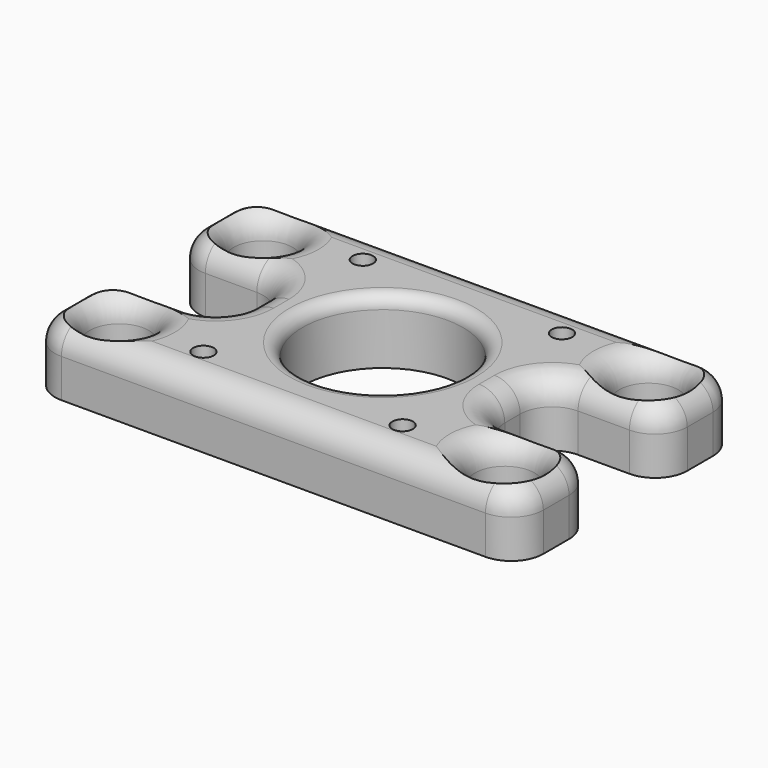
from build123d import *

# Parameters (mm, degrees)
F1_W          = 40
F1_H          = 43
F2_DEPTH      = 10
F3_R          = 12.5
F3_R_2        = 1.6
F4_DEPTH      = 10.001
F5_W          = 18
F5_H          = 15
F5_R          = 2.6
F6_DEPTH      = 10
F7_R          = 5
F8_R          = 4.6
F8_R_2        = 2.6
F9_DEPTH      = 7
F10_T1_DEPTH  = 66
F10_T3_DEPTH  = 3
F10_T5_DEPTH  = 8
F10_T7_DEPTH  = 5
F10_T9_DEPTH  = 8
F10_T11_DEPTH = 5
F10_T22_ANGLE = 90
F10_T24_ANGLE = 90
F10_T26_ANGLE = 90
F10_T28_ANGLE = 90
F10_T30_ANGLE = 90
F10_T32_ANGLE = 90
F10_T34_ANGLE = 90
F10_T36_ANGLE = 90
F10_T38_ANGLE = 90
F10_T40_ANGLE = 90
F10_T42_ANGLE = 90
F10_T44_ANGLE = 90
F11_R         = 2


# Not quite as in the source:
# - a fillet or chamfer that OpenCascade refuses, or shapes differently, is made with other operations: its cross-section is extruded or revolved along the edge and cut away or added
# - a feature names something its author has since deleted; it is built from what else it names


with BuildPart() as f2:
    # F1 (on Top) → F2 (new body)
    with BuildSketch(Plane.XY):
        Rectangle(F1_W, F1_H)
    extrude(amount=F2_DEPTH)

    # F3 (on face) → F4 (cut, through all)
    with BuildSketch(Plane(origin=(0, 0, 0), x_dir=(1, 0, 0), z_dir=(0, 0, -1))):
        with Locations((0, 0.25)):
            Circle(F3_R)
        with Locations((-15.5, -15.25)):
            Circle(F3_R_2)
        with Locations((15.5, -15.25)):
            Circle(F3_R_2)
        with Locations((15.5, 15.75)):
            Circle(F3_R_2)
        with Locations((-15.5, 15.75)):
            Circle(F3_R_2)
    extrude(amount=-F4_DEPTH, mode=Mode.SUBTRACT)

    # F5 (on face) → F6 (join)
    with BuildSketch(Plane(origin=(0, 0, 0), x_dir=(1, 0, 0), z_dir=(0, 0, -1))):
        with Locations((-29, 14)):
            Rectangle(F5_W, F5_H)
        with Locations((-30, 14)):
            Circle(F5_R, mode=Mode.SUBTRACT)
        with Locations((29, 14)):
            Rectangle(F5_W, F5_H)
        with Locations((30, 14)):
            Circle(F5_R, mode=Mode.SUBTRACT)
        with Locations((-29, -14)):
            Rectangle(F5_W, F5_H)
        with Locations((-30, -14)):
            Circle(F5_R, mode=Mode.SUBTRACT)
        with Locations((29, -14)):
            Rectangle(F5_W, F5_H)
        with Locations((30, -14)):
            Circle(F5_R, mode=Mode.SUBTRACT)
    extrude(amount=-F6_DEPTH)

    # F7
    f7_edges = [f2.edges().sort_by_distance(p)[0] for p in [
        (38, -21.5, 5),
        (38, -6.5, 5),
        (-38, -6.5, 5),
        (-38, -21.5, 5),
        (-38, 6.5, 5),
        (-38, 21.5, 5),
        (38, 6.5, 5),
        (38, 21.5, 5),
        (20, 6.5, 5),
        (20, -6.5, 5),
        (-20, 6.5, 5),
        (-20, -6.5, 5),
    ]]
    fillet(f7_edges, radius=F7_R)

    # F8 (on face) → F9 (cut)
    with BuildSketch(Plane.XY.offset(10)):
        with Locations((-30, 14)):
            Circle(F8_R)
        with Locations((-30, 14)):
            Circle(F8_R_2, mode=Mode.SUBTRACT)
        with Locations((-30, -14)):
            Circle(F8_R)
        with Locations((-30, -14)):
            Circle(F8_R_2, mode=Mode.SUBTRACT)
        with Locations((30, 14)):
            Circle(F8_R)
        with Locations((30, 14)):
            Circle(F8_R_2, mode=Mode.SUBTRACT)
        with Locations((30, -14)):
            Circle(F8_R)
        with Locations((30, -14)):
            Circle(F8_R_2, mode=Mode.SUBTRACT)
    extrude(amount=-F9_DEPTH, mode=Mode.SUBTRACT)

    # F10: fillet of radius 4 on 12 edges, made by hand

    # F10_s2 → F10_t1 (cut)
    with BuildSketch(Plane.YZ.offset(-33)):
        with BuildLine():
            ThreePointArc((-17.5, 10), (-20.3284271247, 8.8284271247), (-21.5, 6))
            Line((-21.5, 6), (-21.5, 10))
            Line((-21.5, 10), (-17.5, 10))
        make_face()
        with BuildLine():
            ThreePointArc((21.5, 6), (20.3284271247, 8.8284271247), (17.5, 10))
            Line((17.5, 10), (21.5, 10))
            Line((21.5, 10), (21.5, 6))
        make_face()
    extrude(amount=F10_T1_DEPTH, mode=Mode.SUBTRACT)

    # F10_s4 → F10_t3 (cut)
    with BuildSketch(Plane.XZ.offset(-1.5)):
        with BuildLine():
            ThreePointArc((-16, 10), (-18.8284271247, 8.8284271247), (-20, 6))
            Line((-20, 6), (-20, 10))
            Line((-20, 10), (-16, 10))
        make_face()
        with BuildLine():
            ThreePointArc((16, 10), (18.8284271247, 8.8284271247), (20, 6))
            Line((20, 6), (20, 10))
            Line((20, 10), (16, 10))
        make_face()
    extrude(amount=F10_T3_DEPTH, mode=Mode.SUBTRACT)

    # F10_s6 → F10_t5 (cut)
    with BuildSketch(Plane.YZ.offset(25)):
        with BuildLine():
            ThreePointArc((-10.5, 10), (-7.6715728753, 8.8284271247), (-6.5, 6))
            Line((-6.5, 6), (-6.5, 10))
            Line((-6.5, 10), (-10.5, 10))
        make_face()
        with BuildLine():
            ThreePointArc((10.5, 10), (7.6715728753, 8.8284271247), (6.5, 6))
            Line((6.5, 6), (6.5, 10))
            Line((6.5, 10), (10.5, 10))
        make_face()
    extrude(amount=F10_T5_DEPTH, mode=Mode.SUBTRACT)

    # F10_s8 → F10_t7 (cut)
    with BuildSketch(Plane.XZ.offset(11.5)):
        with BuildLine():
            ThreePointArc((34, 10), (36.8284271247, 8.8284271247), (38, 6))
            Line((38, 6), (38, 10))
            Line((38, 10), (34, 10))
        make_face()
        with BuildLine():
            ThreePointArc((-34, 10), (-36.8284271247, 8.8284271247), (-38, 6))
            Line((-38, 6), (-38, 10))
            Line((-38, 10), (-34, 10))
        make_face()
    extrude(amount=F10_T7_DEPTH, mode=Mode.SUBTRACT)

    # F10_s10 → F10_t9 (cut)
    with BuildSketch(Plane.YZ.offset(-33)):
        with BuildLine():
            ThreePointArc((-10.5, 10), (-7.6715728753, 8.8284271247), (-6.5, 6))
            Line((-6.5, 6), (-6.5, 10))
            Line((-6.5, 10), (-10.5, 10))
        make_face()
        with BuildLine():
            ThreePointArc((10.5, 10), (7.6715728753, 8.8284271247), (6.5, 6))
            Line((6.5, 6), (6.5, 10))
            Line((6.5, 10), (10.5, 10))
        make_face()
    extrude(amount=F10_T9_DEPTH, mode=Mode.SUBTRACT)

    # F10_s12 → F10_t11 (cut)
    with BuildSketch(Plane.XZ.offset(-16.5)):
        with BuildLine():
            ThreePointArc((34, 10), (36.8284271247, 8.8284271247), (38, 6))
            Line((38, 6), (38, 10))
            Line((38, 10), (34, 10))
        make_face()
        with BuildLine():
            ThreePointArc((-34, 10), (-36.8284271247, 8.8284271247), (-38, 6))
            Line((-38, 6), (-38, 10))
            Line((-38, 10), (-34, 10))
        make_face()
    extrude(amount=F10_T11_DEPTH, mode=Mode.SUBTRACT)

    # F10_s13 → F10_t14 (revolve, cut)
    with BuildSketch(Plane.XZ.offset(-14)):
        with BuildLine():
            ThreePointArc((38.6, 10), (35.7715728753, 8.8284271247), (34.6, 6))
            Line((34.6, 6), (34.6, 10))
            Line((34.6, 10), (38.6, 10))
        make_face()
    revolve(axis=Axis((30, 14, 10), (0, 0, 1)), mode=Mode.SUBTRACT)

    # F10_s15 → F10_t16 (revolve, cut)
    with BuildSketch(Plane.XZ.offset(-14)):
        with BuildLine():
            ThreePointArc((-21.4, 10), (-24.2284271247, 8.8284271247), (-25.4, 6))
            Line((-25.4, 6), (-25.4, 10))
            Line((-25.4, 10), (-21.4, 10))
        make_face()
    revolve(axis=Axis((-30, 14, 10), (0, 0, 1)), mode=Mode.SUBTRACT)

    # F10_s17 → F10_t18 (revolve, cut)
    with BuildSketch(Plane.XZ.offset(14)):
        with BuildLine():
            ThreePointArc((-21.4, 10), (-24.2284271247, 8.8284271247), (-25.4, 6))
            Line((-25.4, 6), (-25.4, 10))
            Line((-25.4, 10), (-21.4, 10))
        make_face()
    revolve(axis=Axis((-30, -14, 10), (0, 0, 1)), mode=Mode.SUBTRACT)

    # F10_s19 → F10_t20 (revolve, cut)
    with BuildSketch(Plane.XZ.offset(14)):
        with BuildLine():
            ThreePointArc((38.6, 10), (35.7715728753, 8.8284271247), (34.6, 6))
            Line((34.6, 6), (34.6, 10))
            Line((34.6, 10), (38.6, 10))
        make_face()
    revolve(axis=Axis((30, -14, 10), (0, 0, 1)), mode=Mode.SUBTRACT)

    # F10_s21 → F10_t22 (revolve, cut)
    with BuildSketch(Plane.YZ.offset(-25)):
        with BuildLine():
            ThreePointArc((10.5, 10), (7.6715728753, 8.8284271247), (6.5, 6))
            Line((6.5, 6), (6.5, 10))
            Line((6.5, 10), (10.5, 10))
        make_face()
    revolve(axis=Axis((-25, 1.5, 10), (0, 0, -1)), revolution_arc=F10_T22_ANGLE, mode=Mode.SUBTRACT)

    # F10_s23 → F10_t24 (revolve, cut)
    with BuildSketch(Plane.XZ.offset(-1.5)):
        with BuildLine():
            ThreePointArc((16, 10), (18.8284271247, 8.8284271247), (20, 6))
            Line((20, 6), (20, 10))
            Line((20, 10), (16, 10))
        make_face()
    revolve(axis=Axis((25, 1.5, 10), (0, 0, -1)), revolution_arc=F10_T24_ANGLE, mode=Mode.SUBTRACT)

    # F10_s25 → F10_t26 (revolve, cut)
    with BuildSketch(Plane.XZ.offset(1.5)):
        with BuildLine():
            ThreePointArc((-16, 10), (-18.8284271247, 8.8284271247), (-20, 6))
            Line((-20, 6), (-20, 10))
            Line((-20, 10), (-16, 10))
        make_face()
    revolve(axis=Axis((-25, -1.5, 10), (0, 0, -1)), revolution_arc=F10_T26_ANGLE, mode=Mode.SUBTRACT)

    # F10_s27 → F10_t28 (revolve, cut)
    with BuildSketch(Plane.YZ.offset(25)):
        with BuildLine():
            ThreePointArc((-10.5, 10), (-7.6715728753, 8.8284271247), (-6.5, 6))
            Line((-6.5, 6), (-6.5, 10))
            Line((-6.5, 10), (-10.5, 10))
        make_face()
    revolve(axis=Axis((25, -1.5, 10), (0, 0, -1)), revolution_arc=F10_T28_ANGLE, mode=Mode.SUBTRACT)

    # F10_s29 → F10_t30 (revolve, cut)
    with BuildSketch(Plane.XZ.offset(11.5)):
        with BuildLine():
            ThreePointArc((34, 10), (36.8284271247, 8.8284271247), (38, 6))
            Line((38, 6), (38, 10))
            Line((38, 10), (34, 10))
        make_face()
    revolve(axis=Axis((33, -11.5, 10), (0, 0, 1)), revolution_arc=F10_T30_ANGLE, mode=Mode.SUBTRACT)

    # F10_s31 → F10_t32 (revolve, cut)
    with BuildSketch(Plane.YZ.offset(33)):
        with BuildLine():
            ThreePointArc((-17.5, 10), (-20.3284271247, 8.8284271247), (-21.5, 6))
            Line((-21.5, 6), (-21.5, 10))
            Line((-21.5, 10), (-17.5, 10))
        make_face()
    revolve(axis=Axis((33, -16.5, 10), (0, 0, 1)), revolution_arc=F10_T32_ANGLE, mode=Mode.SUBTRACT)

    # F10_s33 → F10_t34 (revolve, cut)
    with BuildSketch(Plane.YZ.offset(-33)):
        with BuildLine():
            ThreePointArc((-10.5, 10), (-7.6715728753, 8.8284271247), (-6.5, 6))
            Line((-6.5, 6), (-6.5, 10))
            Line((-6.5, 10), (-10.5, 10))
        make_face()
    revolve(axis=Axis((-33, -11.5, 10), (0, 0, 1)), revolution_arc=F10_T34_ANGLE, mode=Mode.SUBTRACT)

    # F10_s35 → F10_t36 (revolve, cut)
    with BuildSketch(Plane.XZ.offset(16.5)):
        with BuildLine():
            ThreePointArc((-34, 10), (-36.8284271247, 8.8284271247), (-38, 6))
            Line((-38, 6), (-38, 10))
            Line((-38, 10), (-34, 10))
        make_face()
    revolve(axis=Axis((-33, -16.5, 10), (0, 0, 1)), revolution_arc=F10_T36_ANGLE, mode=Mode.SUBTRACT)

    # F10_s37 → F10_t38 (revolve, cut)
    with BuildSketch(Plane.YZ.offset(33)):
        with BuildLine():
            ThreePointArc((10.5, 10), (7.6715728753, 8.8284271247), (6.5, 6))
            Line((6.5, 6), (6.5, 10))
            Line((6.5, 10), (10.5, 10))
        make_face()
    revolve(axis=Axis((33, 11.5, 10), (0, 0, 1)), revolution_arc=F10_T38_ANGLE, mode=Mode.SUBTRACT)

    # F10_s39 → F10_t40 (revolve, cut)
    with BuildSketch(Plane.YZ.offset(33)):
        with BuildLine():
            ThreePointArc((21.5, 6), (20.3284271247, 8.8284271247), (17.5, 10))
            Line((17.5, 10), (21.5, 10))
            Line((21.5, 10), (21.5, 6))
        make_face()
    revolve(axis=Axis((33, 16.5, 10), (0, 0, -1)), revolution_arc=F10_T40_ANGLE, mode=Mode.SUBTRACT)

    # F10_s41 → F10_t42 (revolve, cut)
    with BuildSketch(Plane.XZ.offset(-11.5)):
        with BuildLine():
            ThreePointArc((-34, 10), (-36.8284271247, 8.8284271247), (-38, 6))
            Line((-38, 6), (-38, 10))
            Line((-38, 10), (-34, 10))
        make_face()
    revolve(axis=Axis((-33, 11.5, 10), (0, 0, 1)), revolution_arc=F10_T42_ANGLE, mode=Mode.SUBTRACT)

    # F10_s43 → F10_t44 (revolve, cut)
    with BuildSketch(Plane.YZ.offset(-33)):
        with BuildLine():
            ThreePointArc((21.5, 6), (20.3284271247, 8.8284271247), (17.5, 10))
            Line((17.5, 10), (21.5, 10))
            Line((21.5, 10), (21.5, 6))
        make_face()
    revolve(axis=Axis((-33, 16.5, 10), (0, 0, 1)), revolution_arc=F10_T44_ANGLE, mode=Mode.SUBTRACT)

    # F11
    f11_edges = [f2.edges().sort_by_distance(p)[0] for p in [
        (-12.5, -0.25, 10),
    ]]
    fillet(f11_edges, radius=F11_R)


solid = f2.part
